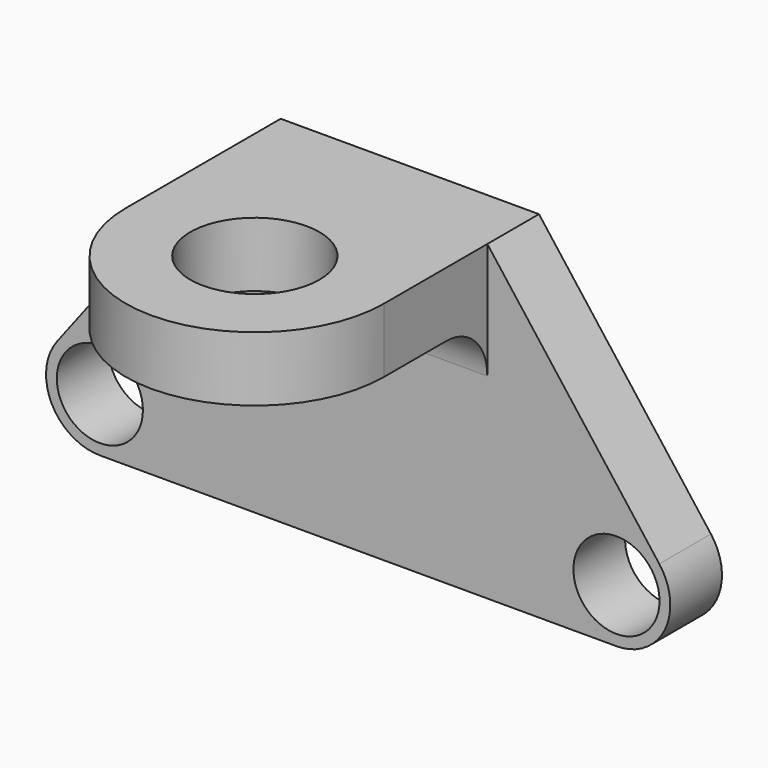
from build123d import *

# Parameters (mm, degrees)
F0_R     = 10
F1_DEPTH = 15
F3_R     = 15
F4_DEPTH = 15
F5_R     = 12


# Not quite as in the source:
# - ends of sketch curves that miss each other by under 0.0002 mm in the source are joined


with BuildPart() as f1:
    # F0 (on Front) → F1 (new body)
    with BuildSketch(Plane.XZ):
        with BuildLine():
            Line((-30, 24.9995148627), (-69.9428552721, -27.4248908346))
            ThreePointArc((-69.9428552721, -27.4248908346), (-71.2014492094, -40.5482356371), (-60, -47.5004851373))
            Line((-60, -47.5004851373), (60, -47.5004851373))
            ThreePointArc((60, -47.5004851373), (71.2014492094, -40.5482356371), (69.9428552721, -27.4248908346))
            Line((69.9428552721, -27.4248908346), (30, 24.9995148627))
            Line((30, 24.9995148627), (0, 24.9995148627))
            Line((0, 24.9995148627), (-30, 24.9995148627))
        make_face()
        with Locations((-60, -35.0004851373)):
            Circle(F0_R, mode=Mode.SUBTRACT)
        with Locations((60, -35.0004851373)):
            Circle(F0_R, mode=Mode.SUBTRACT)
    extrude(amount=F1_DEPTH)

    # F3 (on offset) → F4 (join)
    with BuildSketch(Plane.XY.offset(24.9995148627)):
        with BuildLine():
            Line((-30, -14.9999307469), (-30, -45.0000600332))
            ThreePointArc((-30, -45.0000600332), (2.21189e-05, -75), (30, -45.0000157953))
            Line((30, -45.0000157953), (30, -14.9999307469))
            Line((30, -14.9999307469), (30, 0))
            Line((30, 0), (-30, 0))
            Line((-30, 0), (-30, -14.9999307469))
        make_face()
        with Locations((0, -45)):
            Circle(F3_R, mode=Mode.SUBTRACT)
    extrude(amount=-F4_DEPTH)

    # F5
    f5_edges = [f1.edges().sort_by_distance(p)[0] for p in [
        (0, -15, 9.999515),
    ]]
    fillet(f5_edges, radius=F5_R)


solid = f1.part
